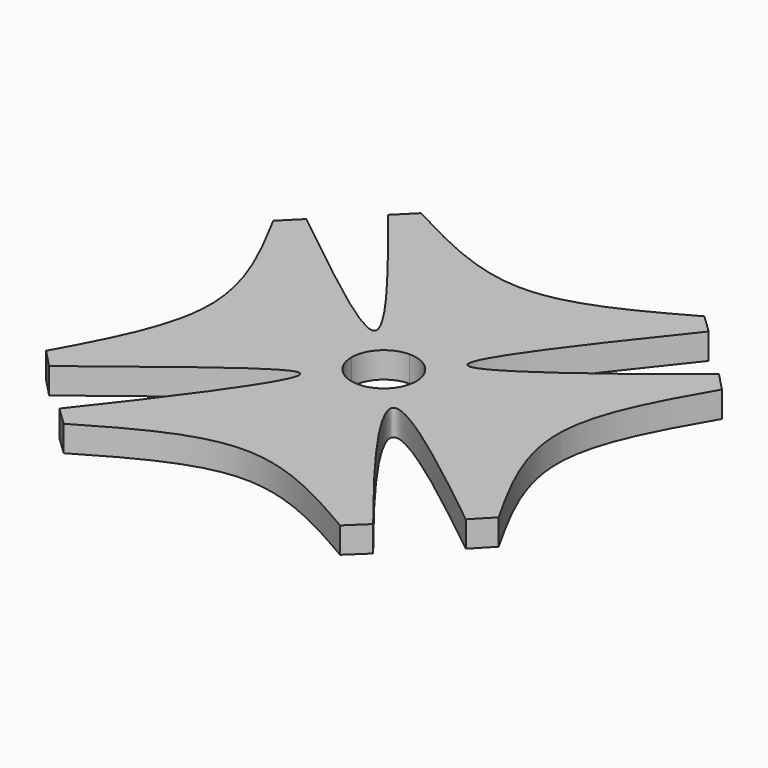
from build123d import *

# Parameters (mm, degrees)
F2_DEPTH = 5.08
F3_DEPTH = 5.08


with BuildPart() as f2:
    # F1 (on Top) → F2 (new body)
    with BuildSketch(Plane.XY):
        with BuildLine():
            add(Edge.make_bspline(
                [(-40.3796768019, 31.486727974), (-25.4125832668, 19.5130531459), (4.2719382832, -4.2719382832), (-19.5130531459, 25.4125832668), (-31.486727974, 40.3796768019)],
                knots=[0, 0, 0, 0, 0.5, 1, 1, 1, 1], degree=3))
            Line((-40.3796768019, 31.486727974), (-43.9717792504, 27.8946255256))
            add(Edge.make_bspline(
                [(-43.9717792504, 27.8946255256), (-39.0223614388, 18.5744758569), (-29.1485977035, -0.0186111101), (-39.1966306531, -18.3497362141), (-44.207889928, -27.4920251734)],
                knots=[0, 0, 0, 0, 0.5012696216, 1, 1, 1, 1], degree=3))
            Line((-44.207889928, -27.4920251734), (-40.688852268, -31.1557355805))
            add(Edge.make_bspline(
                [(-40.688852268, -31.1557355805), (-25.5161789229, -19.5156604784), (3.9712190003, 4.6498080898), (-18.7967685048, -26.1767940312), (-30.6525350904, -41.1896309485)],
                knots=[0, 0, 0, 0, 0.4995827747, 1, 1, 1, 1], degree=3))
            Line((-30.6525350904, -41.1896309485), (-26.9813712251, -44.7008922424))
            add(Edge.make_bspline(
                [(-26.9813712251, -44.7008922424), (-17.9946084514, -39.4329857114), (-0.010494669, -28.8909659837), (18.0580501184, -39.3550908644), (27.0976414843, -44.5902337071)],
                knots=[0, 0, 0, 0, 0.4997056226, 1, 1, 1, 1], degree=3))
            Line((27.0976414843, -44.5902337071), (30.7701121053, -41.0803391876))
            add(Edge.make_bspline(
                [(30.7701121053, -41.0803391876), (18.791953604, -26.107641061), (-4.1552313798, 4.3732948199), (25.8949419877, -19.0260044621), (40.8564309314, -30.995195617)],
                knots=[0, 0, 0, 0, 0.5001872305, 1, 1, 1, 1], degree=3))
            Line((40.8564309314, -30.995195617), (44.3699422534, -27.3261850978))
            add(Edge.make_bspline(
                [(44.5902337071, 27.0976414843), (39.403270189, 18.0788208761), (29.0172364099, 0.0201290891), (39.2483982347, -18.2036660263), (44.3699422534, -27.3261850978)],
                knots=[0, 0, 0, 0, 0.4994171624, 1, 1, 1, 1], degree=3))
            Line((44.5902337071, 27.0976414843), (41.0803391876, 30.7701121053))
            add(Edge.make_bspline(
                [(30.995195617, 40.8564309314), (19.0260044621, 25.8949419877), (-4.3732948199, -4.1552313798), (26.107641061, 18.791953604), (41.0803391876, 30.7701121053)],
                knots=[0, 0, 0, 0, 0.4998127695, 1, 1, 1, 1], degree=3))
            Line((30.995195617, 40.8564309314), (27.3261850978, 44.3699422534))
            add(Edge.make_bspline(
                [(-27.8946255256, 43.9717792504), (-18.5644448783, 39.0204369591), (0.0328141053, 29.1512395247), (18.2489978621, 39.3085295686), (27.3261850978, 44.3699422534)],
                knots=[0, 0, 0, 0, 0.5016965487, 1, 1, 1, 1], degree=3))
            Line((-27.8946255256, 43.9717792504), (-31.486727974, 40.3796768019))
        make_face()
    extrude(amount=-F2_DEPTH)

    # F0 (on Top) → F3 (cut, through all)
    with BuildSketch(Plane.XY):
        with BuildLine():
            ThreePointArc((0, -6.35), (4.4901280605, -4.4901280605), (6.35, 0))
            ThreePointArc((6.35, 0), (4.4901280605, 4.4901280605), (0, 6.35))
            ThreePointArc((0, 6.35), (-4.4901280605, 4.4901280605), (-6.35, 0))
            ThreePointArc((-6.35, 0), (-4.4901280605, -4.4901280605), (0, -6.35))
        make_face()
    extrude(amount=-F3_DEPTH, mode=Mode.SUBTRACT)


solid = f2.part
